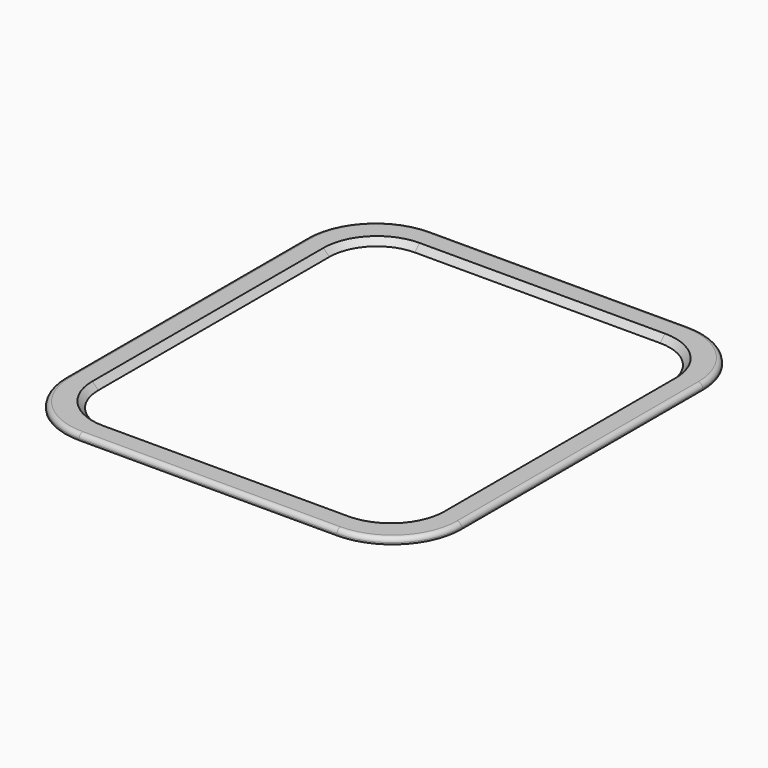
from build123d import *

# Parameters (mm, degrees)
F2_DEPTH     = 1.2065
F3_DEPTH     = 1.2075
F4_R         = 0.8763
F5_T1_DEPTH  = 58.42
F5_T3_DEPTH  = 49.6062
F5_T6_ANGLE  = 90
F5_T8_ANGLE  = 90
F5_T10_ANGLE = 90
F5_T12_ANGLE = 90


# Not quite as in the source:
# - a fillet or chamfer that OpenCascade refuses, or shapes differently, is made with other operations: its cross-section is extruded or revolved along the edge and cut away or added


with BuildPart() as f2:
    # F0 (on Top) → F2 (new body)
    with BuildSketch(Plane.XY):
        with BuildLine():
            ThreePointArc((40.0431, 30.4673), (35.9476619893, 40.3545619893), (26.0604, 44.45))
            Line((26.0604, 44.45), (-26.0604, 44.45))
            ThreePointArc((-26.0604, 44.45), (-35.9476619893, 40.3545619893), (-40.0431, 30.4673))
            Line((-40.0431, 30.4673), (-40.0431, -30.4673))
            ThreePointArc((-40.0431, -30.4673), (-35.9476619893, -40.3545619893), (-26.0604, -44.45))
            Line((-26.0604, -44.45), (26.0604, -44.45))
            ThreePointArc((26.0604, -44.45), (35.9476619893, -40.3545619893), (40.0431, -30.4673))
            Line((40.0431, -30.4673), (40.0431, 30.4673))
        make_face()
    extrude(amount=F2_DEPTH)

    # F1 (on Top) + F2_face (on face) → F3 (cut, through all)
    with BuildSketch(Plane.XY):
        with BuildLine():
            ThreePointArc((34.3281, 29.21), (31.5382920908, 35.9451920908), (24.8031, 38.735))
            Line((24.8031, 38.735), (-24.8031, 38.735))
            ThreePointArc((-24.8031, 38.735), (-31.5382920908, 35.9451920908), (-34.3281, 29.21))
            Line((-34.3281, 29.21), (-34.3281, -29.21))
            ThreePointArc((-34.3281, -29.21), (-31.5382920908, -35.9451920908), (-24.8031, -38.735))
            Line((-24.8031, -38.735), (24.8031, -38.735))
            ThreePointArc((24.8031, -38.735), (31.5382920908, -35.9451920908), (34.3281, -29.21))
            Line((34.3281, -29.21), (34.3281, 29.21))
        make_face()
    with BuildSketch(Plane.XY.offset(1.2065)):
        with BuildLine():
            ThreePointArc((40.0431, 30.4673), (35.9476619893, 40.3545619893), (26.0604, 44.45))
            Line((26.0604, 44.45), (-26.0604, 44.45))
            ThreePointArc((-26.0604, 44.45), (-35.9476619893, 40.3545619893), (-40.0431, 30.4673))
            Line((-40.0431, 30.4673), (-40.0431, -30.4673))
            ThreePointArc((-40.0431, -30.4673), (-35.9476619893, -40.3545619893), (-26.0604, -44.45))
            Line((-26.0604, -44.45), (26.0604, -44.45))
            ThreePointArc((26.0604, -44.45), (35.9476619893, -40.3545619893), (40.0431, -30.4673))
            Line((40.0431, -30.4673), (40.0431, 30.4673))
        make_face()
    extrude(amount=F3_DEPTH, mode=Mode.SUBTRACT)

    # F4
    f4_edges = [f2.edges().sort_by_distance(p)[0] for p in [
        (-40.0431, 0, 1.2065),
    ]]
    fillet(f4_edges, radius=F4_R)

    # F5: chamfer of 1.27 on 1 edges, made by hand

    # F5_s2 → F5_t1 (cut)
    with BuildSketch(Plane.XZ.offset(-29.21)):
        Polygon((-35.5981, 1.2065), (-34.3281, -0.0635), (-34.3281, 1.2065), align=None)
        Polygon((35.5981, 1.2065), (34.3281, -0.0635), (34.3281, 1.2065), align=None)
    extrude(amount=F5_T1_DEPTH, mode=Mode.SUBTRACT)

    # F5_s4 → F5_t3 (cut)
    with BuildSketch(Plane.YZ.offset(-24.8031)):
        Polygon((-40.005, 1.2065), (-38.735, -0.0635), (-38.735, 1.2065), align=None)
        Polygon((40.005, 1.2065), (38.735, -0.0635), (38.735, 1.2065), align=None)
    extrude(amount=F5_T3_DEPTH, mode=Mode.SUBTRACT)

    # F5_s5 → F5_t6 (revolve, cut)
    with BuildSketch(Plane.XZ.offset(-29.21)):
        Polygon((-35.5981, 1.2065), (-34.3281, -0.0635), (-34.3281, 1.2065), align=None)
    revolve(axis=Axis((-24.8031, 29.21, 1.2065), (0, 0, -1)), revolution_arc=F5_T6_ANGLE, mode=Mode.SUBTRACT)

    # F5_s7 → F5_t8 (revolve, cut)
    with BuildSketch(Plane.YZ.offset(-24.8031)):
        Polygon((-40.005, 1.2065), (-38.735, -0.0635), (-38.735, 1.2065), align=None)
    revolve(axis=Axis((-24.8031, -29.21, 1.2065), (0, 0, -1)), revolution_arc=F5_T8_ANGLE, mode=Mode.SUBTRACT)

    # F5_s9 → F5_t10 (revolve, cut)
    with BuildSketch(Plane.XZ.offset(29.21)):
        Polygon((35.5981, 1.2065), (34.3281, -0.0635), (34.3281, 1.2065), align=None)
    revolve(axis=Axis((24.8031, -29.21, 1.2065), (0, 0, -1)), revolution_arc=F5_T10_ANGLE, mode=Mode.SUBTRACT)

    # F5_s11 → F5_t12 (revolve, cut)
    with BuildSketch(Plane.YZ.offset(24.8031)):
        Polygon((40.005, 1.2065), (38.735, -0.0635), (38.735, 1.2065), align=None)
    revolve(axis=Axis((24.8031, 29.21, 1.2065), (0, 0, -1)), revolution_arc=F5_T12_ANGLE, mode=Mode.SUBTRACT)


solid = f2.part
